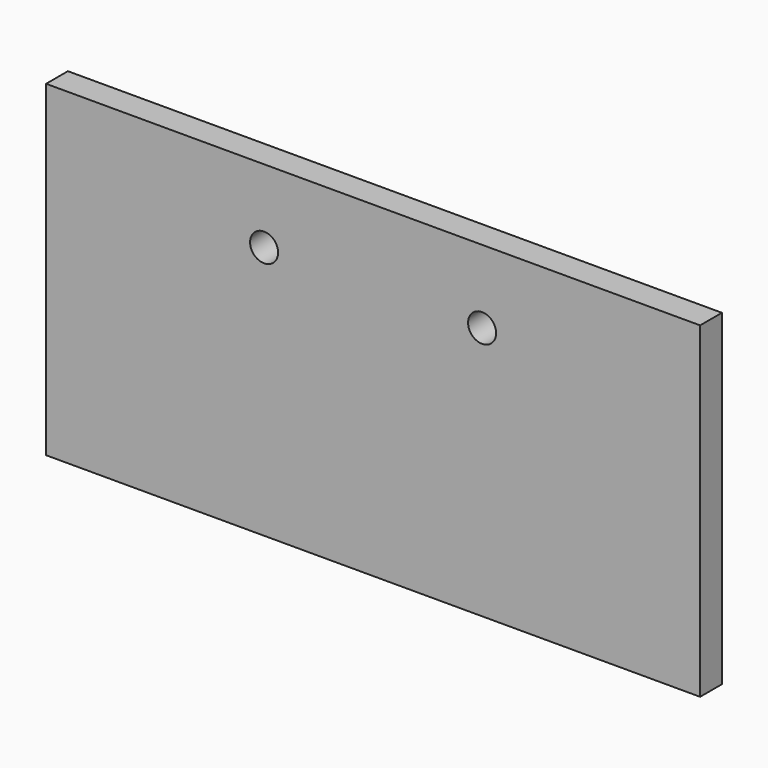
from build123d import *

# Parameters (mm, degrees)
F0_W     = 152.4
F0_H     = 6.35
F1_DEPTH = 76.2
F2_R     = 3.2639
F3_DEPTH = 6.351


# Not quite as in the source:
# - a feature names something its author has since deleted; it is built from what else it names


with BuildPart() as f1:
    # F0 (on Top) → F1 (new body)
    with BuildSketch(Plane.XY):
        with Locations((76.2, 51.9430038067)):
            Rectangle(F0_W, F0_H)
    extrude(amount=F1_DEPTH)

    # F2 (on face) → F3 (cut, through all)
    with BuildSketch(Plane.XZ.offset(-48.7680038067)):
        with Locations((101.6, 59.1464154422)):
            Circle(F2_R)
        with Locations((50.8, 59.1464154422)):
            Circle(F2_R)
    extrude(amount=-F3_DEPTH, mode=Mode.SUBTRACT)


solid = f1.part
